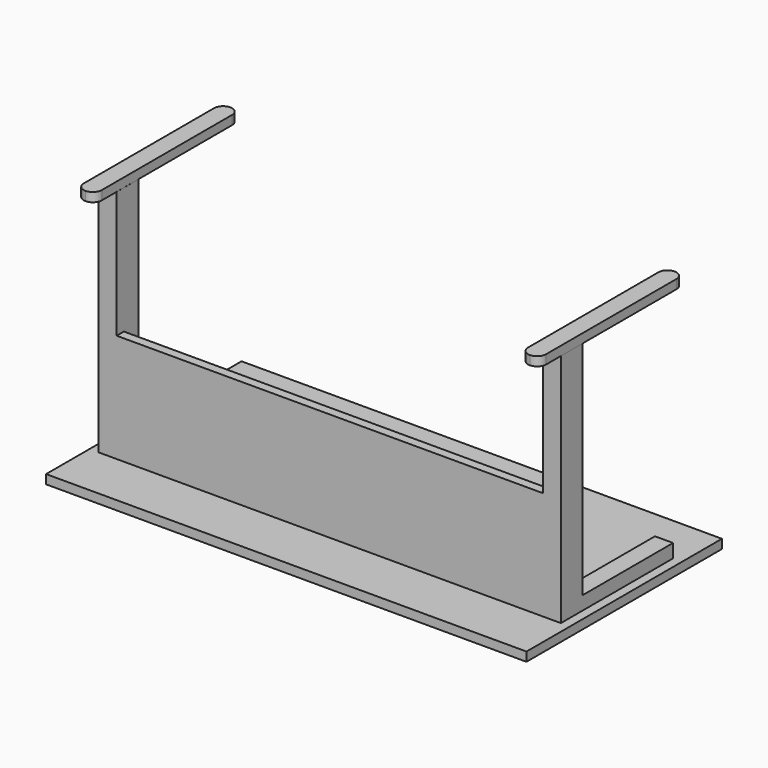
from build123d import *

# Parameters (mm, degrees)
F1_DEPTH = 25.4
F2_W     = 50.8
F2_H     = 317.5
F3_DEPTH = 38.1
F4_W     = 50.8
F4_H     = 76.2
F5_DEPTH = 660.4
F7_DEPTH = 25.4
F8_W     = 1196.34
F8_H     = 25.4
F9_DEPTH = 304.8


# Not quite as in the source:
# - a feature names something its author has since deleted; it is built from what else it names


with BuildPart() as f1:
    # F0 (on Top) → F1 (new body)
    with BuildSketch(Plane.XY):
        Polygon((-674.37, -342.9), (674.37, -342.9), (674.37, 342.9), (-674.37, 342.9), (-674.37, -114.3), align=None)
    extrude(amount=F1_DEPTH)

    # F2 (on face) → F3 (join)
    with BuildSketch(Plane.XY.offset(25.4)):
        with Locations((-623.57, 44.45)):
            Rectangle(F2_W, F2_H)
        with Locations((623.57, 44.45)):
            Rectangle(F2_W, F2_H)
    extrude(amount=F3_DEPTH)

    # F4 (on face) → F5 (join)
    with BuildSketch(Plane.XY.offset(25.4)):
        with Locations((-623.57, -152.4)):
            Rectangle(F4_W, F4_H)
        with Locations((623.57, -152.4)):
            Rectangle(F4_W, F4_H)
    extrude(amount=F5_DEPTH)

    # F6 (on face) → F7 (join)
    with BuildSketch(Plane.XY.offset(685.8)):
        with BuildLine():
            ThreePointArc((-623.6857005119, -267.7317205817), (-605.7251882698, -260.2922328238), (-598.2857005119, -242.3317205817))
            Line((-598.2857005119, -242.3317205817), (-598.2857005119, 214.8682794183))
            ThreePointArc((-598.2857005119, 214.8682794183), (-605.7251882698, 232.8287916605), (-623.6857005119, 240.2682794183))
            ThreePointArc((-623.6857005119, 240.2682794183), (-641.6462127541, 232.8287916605), (-649.0857005119, 214.8682794183))
            Line((-649.0857005119, 214.8682794183), (-649.0857005119, -242.3317205817))
            ThreePointArc((-649.0857005119, -242.3317205817), (-641.6462127541, -260.2922328238), (-623.6857005119, -267.7317205817))
        make_face()
        with BuildLine():
            ThreePointArc((623.6857005119, -267.7317205817), (641.6462127541, -260.2922328238), (649.0857005119, -242.3317205817))
            Line((649.0857005119, -242.3317205817), (649.0857005119, 214.8682794183))
            ThreePointArc((649.0857005119, 214.8682794183), (641.6462127541, 232.8287916605), (623.6857005119, 240.2682794183))
            ThreePointArc((623.6857005119, 240.2682794183), (605.7251882698, 232.8287916605), (598.2857005119, 214.8682794183))
            Line((598.2857005119, 214.8682794183), (598.2857005119, -242.3317205817))
            ThreePointArc((598.2857005119, -242.3317205817), (605.7251882698, -260.2922328238), (623.6857005119, -267.7317205817))
        make_face()
    extrude(amount=F7_DEPTH)

    # F8 (on face) → F9 (join)
    with BuildSketch(Plane.XY.offset(25.4)):
        with Locations((0, -177.8)):
            Rectangle(F8_W, F8_H)
    extrude(amount=F9_DEPTH)


solid = f1.part
